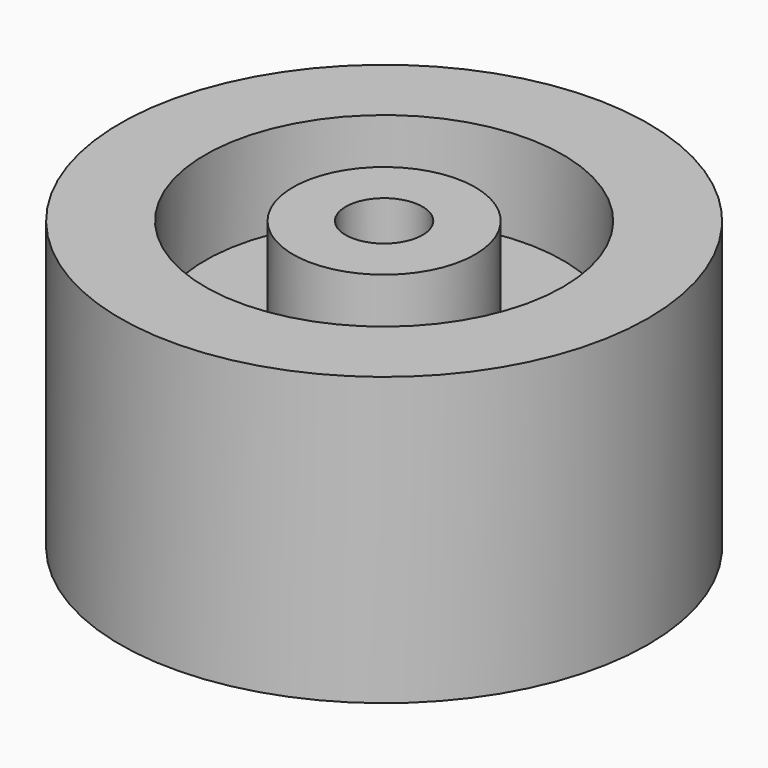
from build123d import *

# Parameters (mm, degrees)
F4_D     = 4.2
F4_DEPTH = 27.8
F4_TIP   = 1.2618073


# Not quite as in the source:
# - a feature of the source that left no trace in its solid (it failed there, or was rolled back) is left out


with BuildPart() as f1:
    # F0 (on Front) → F1 (revolve)
    with BuildSketch(Plane.XZ):
        Polygon((4.9784, 0), (0, 0), (0, -15.6972), (14.4272, -15.6972), (14.4272, 0), (9.779, 0), (9.779, -5.08), (4.9784, -5.08), align=None)
    revolve(axis=Axis((0, 0, -7.8486), (0, 0, 1)))

    # F4
    with Locations(Plane(origin=(0, 0, -15.6972), x_dir=(1, 0, 0), z_dir=(0, 0, -1))):
        with Locations((0, 0)):
            Hole(F4_D / 2, depth=F4_DEPTH)
            with Locations((0, 0, -(F4_DEPTH + F4_TIP / 2))):  # 118° drill point
                Cone(0, F4_D / 2, F4_TIP, mode=Mode.SUBTRACT)


solid = f1.part
